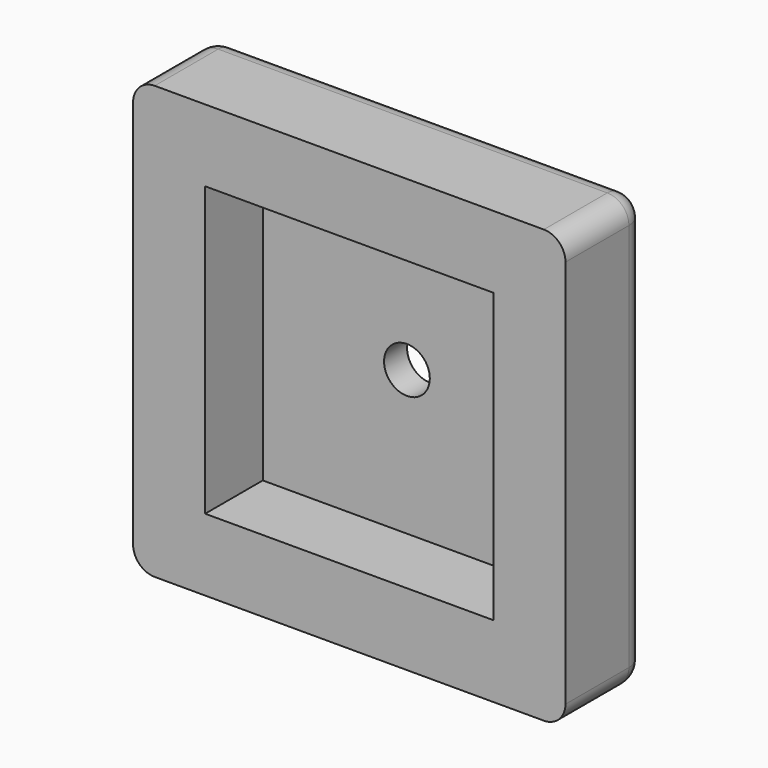
from build123d import *

# Parameters (mm, degrees)
F0_W     = 60
F0_H     = 60
F0_W_2   = 40
F0_H_2   = 40
F1_DEPTH = 14
F0_R     = 3.175
F2_DEPTH = 4
F3_R     = 3


# Not quite as in the source:
# - a feature names something its author has since deleted; it is built from what else it names


with BuildPart() as f1:
    # F0 (on Front) → F1 (new body)
    with BuildSketch(Plane.XZ):
        with Locations((30, 30)):
            Rectangle(F0_W, F0_H)
        with Locations((30, 30)):
            Rectangle(F0_W_2, F0_H_2, mode=Mode.SUBTRACT)
    extrude(amount=F1_DEPTH)

    # F0 (on Front) → F2 (join)
    with BuildSketch(Plane.XZ):
        with Locations((30, 30)):
            Rectangle(F0_W_2, F0_H_2)
        with Locations((30, 30)):
            Circle(F0_R, mode=Mode.SUBTRACT)
    extrude(amount=F2_DEPTH)

    # F3
    f3_edges = [f1.edges().sort_by_distance(p)[0] for p in [
        (0, -7, 0),
        (0, -7, 60),
        (60, -7, 60),
        (60, -7, 0),
        (60, 0, 30),
        (30, 0, 60),
        (0, 0, 30),
        (30, 0, 0),
    ]]
    fillet(f3_edges, radius=F3_R)


solid = f1.part
